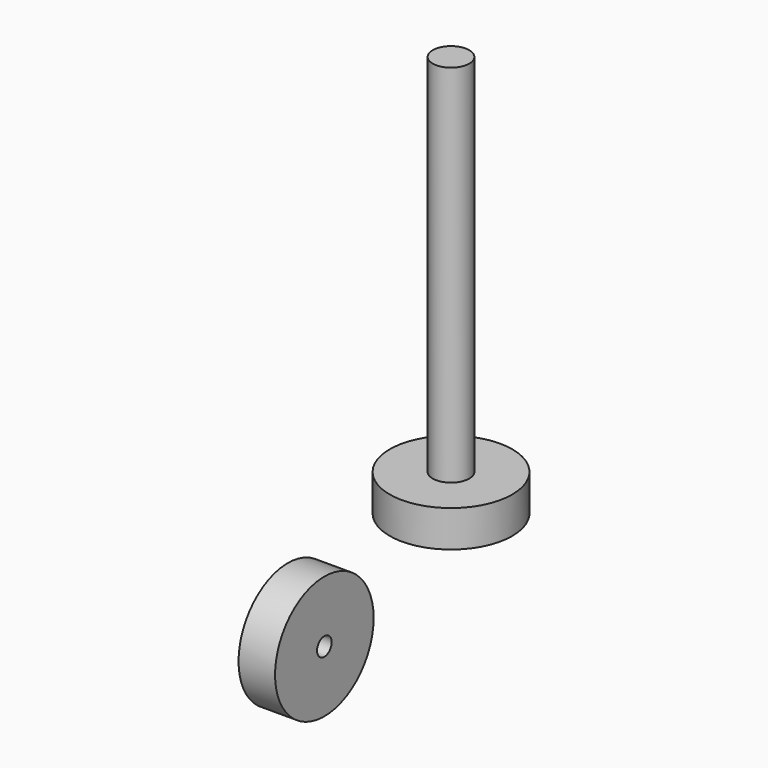
from build123d import *

# Parameters (mm, degrees)
F0_R     = 42.6042021987
F1_DEPTH = 25.4
F2_R     = 42.8158000792
F3_DEPTH = 25.4
F4_R     = 12.7
F5_DEPTH = 254
F6_R     = 6.35
F7_DEPTH = 25.4


with BuildPart() as f1:
    # F0 (on Top) → F1 (new body)
    with BuildSketch(Plane.XY):
        Circle(F0_R)
    extrude(amount=F1_DEPTH)


with BuildPart() as f3:
    # F2 (on Right) → F3 (new body)
    with BuildSketch(Plane.YZ):
        with Locations((-141.8243199587, -15.5356675386)):
            Circle(F2_R)
    extrude(amount=F3_DEPTH)

    # F6 (on face) → F7 (cut)
    with BuildSketch(Plane(origin=(0, 0, 0), x_dir=(0, -1, 0), z_dir=(-1, 0, 0))):
        with Locations((141.8243199587, -15.5356675386)):
            Circle(F6_R)
    extrude(amount=-F7_DEPTH, mode=Mode.SUBTRACT)


with BuildPart() as f5:
    # F4 (on face) → F5 (new body)
    with BuildSketch(Plane.XY.offset(25.4)):
        Circle(F4_R)
    extrude(amount=F5_DEPTH)


solid = Compound([f1.part, f3.part, f5.part])
